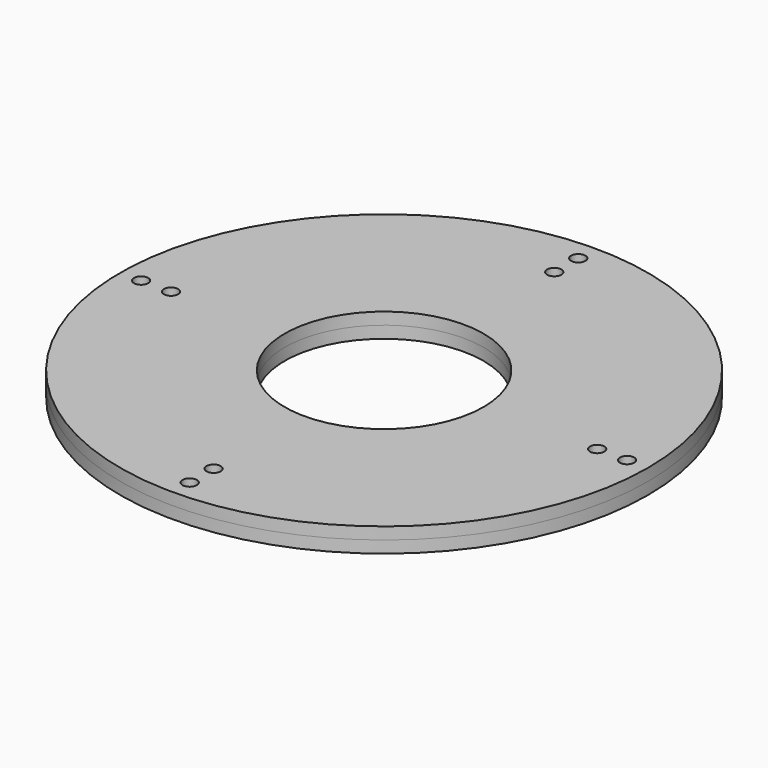
from build123d import *

# Parameters (mm, degrees)
F0_R     = 69.85
F0_R_2   = 1.8923
F0_R_3   = 26.3144
F1_DEPTH = 3.175
F3_DEPTH = 3.175


# Not quite as in the source:
# - a feature names something its author has since deleted; it is built from what else it names


with BuildPart() as f1:
    # F0 (on Top) → F1 (new body)
    with BuildSketch(Plane.XY):
        Circle(F0_R)
        with Locations((0, -64.3023502119)):
            Circle(F0_R_2, mode=Mode.SUBTRACT)
        with Locations((0, -56.38329491)):
            Circle(F0_R_2, mode=Mode.SUBTRACT)
        with Locations((-64.3023502119, 0)):
            Circle(F0_R_2, mode=Mode.SUBTRACT)
        with Locations((-56.38329491, 0)):
            Circle(F0_R_2, mode=Mode.SUBTRACT)
        Circle(F0_R_3, mode=Mode.SUBTRACT)
        with Locations((56.38329491, 0)):
            Circle(F0_R_2, mode=Mode.SUBTRACT)
        with Locations((64.3023502119, 0)):
            Circle(F0_R_2, mode=Mode.SUBTRACT)
        with Locations((0, 56.2991)):
            Circle(F0_R_2, mode=Mode.SUBTRACT)
        with Locations((0, 64.2239)):
            Circle(F0_R_2, mode=Mode.SUBTRACT)
    extrude(amount=-F1_DEPTH)


with BuildPart() as f3:
    # F0 (on Top) → F3 (new body)
    with BuildSketch(Plane.XY):
        Circle(F0_R)
        with Locations((0, -64.3023502119)):
            Circle(F0_R_2, mode=Mode.SUBTRACT)
        with Locations((0, -56.38329491)):
            Circle(F0_R_2, mode=Mode.SUBTRACT)
        with Locations((-64.3023502119, 0)):
            Circle(F0_R_2, mode=Mode.SUBTRACT)
        with Locations((-56.38329491, 0)):
            Circle(F0_R_2, mode=Mode.SUBTRACT)
        Circle(F0_R_3, mode=Mode.SUBTRACT)
        with Locations((56.38329491, 0)):
            Circle(F0_R_2, mode=Mode.SUBTRACT)
        with Locations((64.3023502119, 0)):
            Circle(F0_R_2, mode=Mode.SUBTRACT)
        with Locations((0, 56.2991)):
            Circle(F0_R_2, mode=Mode.SUBTRACT)
        with Locations((0, 64.2239)):
            Circle(F0_R_2, mode=Mode.SUBTRACT)
    extrude(amount=F3_DEPTH)


solid = Compound([f1.part, f3.part])
